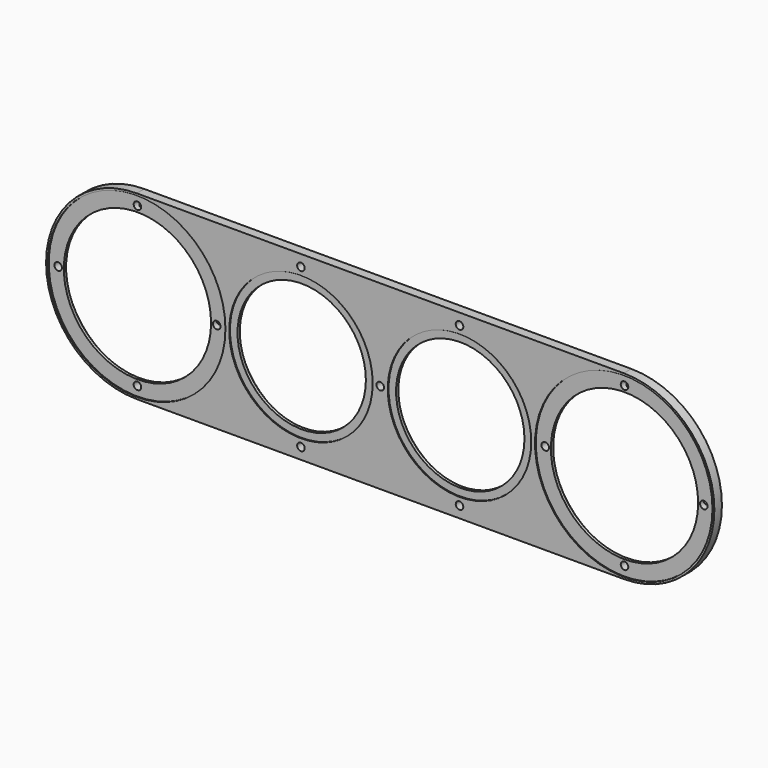
from build123d import *

# Parameters (mm, degrees)
F0_R     = 2
F0_R_2   = 39
F0_R_3   = 34
F1_DEPTH = 5
F2_R     = 38
F2_R_2   = 47
F3_DEPTH = 0.5


# Not quite as in the source:
# - a fillet or chamfer that OpenCascade refuses, or shapes differently, is made with other operations: its cross-section is extruded or revolved along the edge and cut away or added


with BuildPart() as f1:
    # F0 (on Front) → F1 (new body)
    with BuildSketch(Plane.XZ):
        with BuildLine():
            ThreePointArc((129, -48), (177, 0), (129, 48))
            Line((129, 48), (0, 48))
            Line((0, 48), (-129, 48))
            ThreePointArc((-129, 48), (-177, 0), (-129, -48))
            Line((-129, -48), (0, -48))
            Line((0, -48), (129, -48))
        make_face()
        with Locations((-129, -42)):
            Circle(F0_R, mode=Mode.SUBTRACT)
        with Locations((-42, -42)):
            Circle(F0_R, mode=Mode.SUBTRACT)
        with Locations((42, -42)):
            Circle(F0_R, mode=Mode.SUBTRACT)
        with Locations((129, -42)):
            Circle(F0_R, mode=Mode.SUBTRACT)
        with Locations((-171, 0)):
            Circle(F0_R, mode=Mode.SUBTRACT)
        with Locations((-129, 0)):
            Circle(F0_R_2, mode=Mode.SUBTRACT)
        with Locations((-87, 0)):
            Circle(F0_R, mode=Mode.SUBTRACT)
        with Locations((-42, 0)):
            Circle(F0_R_3, mode=Mode.SUBTRACT)
        with Locations((-129, 42)):
            Circle(F0_R, mode=Mode.SUBTRACT)
        with Locations((-42, 42)):
            Circle(F0_R, mode=Mode.SUBTRACT)
        Circle(F0_R, mode=Mode.SUBTRACT)
        with Locations((42, 0)):
            Circle(F0_R_3, mode=Mode.SUBTRACT)
        with Locations((87, 0)):
            Circle(F0_R, mode=Mode.SUBTRACT)
        with Locations((129, 0)):
            Circle(F0_R_2, mode=Mode.SUBTRACT)
        with Locations((171, 0)):
            Circle(F0_R, mode=Mode.SUBTRACT)
        with Locations((42, 42)):
            Circle(F0_R, mode=Mode.SUBTRACT)
        with Locations((129, 42)):
            Circle(F0_R, mode=Mode.SUBTRACT)
    extrude(amount=F1_DEPTH)

    # F2 (on face) → F3 (cut)
    with BuildSketch(Plane.XZ.offset(5)):
        with Locations((42, 0)):
            Circle(F2_R)
        with Locations((-42, 0)):
            Circle(F2_R)
        with Locations((129, 0)):
            Circle(F2_R_2)
        with Locations((-129, 0)):
            Circle(F2_R_2)
    extrude(amount=-F3_DEPTH, mode=Mode.SUBTRACT)

    # F4: chamfer of 3 on 4 edges, made by hand

    # F4_s1 → F4_t2 (revolve, cut)
    with BuildSketch(Plane.XY):
        Polygon((-87, 0), (-90, -3), (-90, 0), align=None)
    revolve(axis=Axis((-129, 0, 0), (0, -1, 0)), mode=Mode.SUBTRACT)

    # F4_s3 → F4_t4 (revolve, cut)
    with BuildSketch(Plane.XY):
        Polygon((-5, 0), (-8, -3), (-8, 0), align=None)
    revolve(axis=Axis((-42, 0, 0), (0, -1, 0)), mode=Mode.SUBTRACT)

    # F4_s5 → F4_t6 (revolve, cut)
    with BuildSketch(Plane.XY):
        Polygon((79, 0), (76, -3), (76, 0), align=None)
    revolve(axis=Axis((42, 0, 0), (0, -1, 0)), mode=Mode.SUBTRACT)

    # F4_s7 → F4_t8 (revolve, cut)
    with BuildSketch(Plane.XY):
        Polygon((171, 0), (168, -3), (168, 0), align=None)
    revolve(axis=Axis((129, 0, 0), (0, -1, 0)), mode=Mode.SUBTRACT)


solid = f1.part
